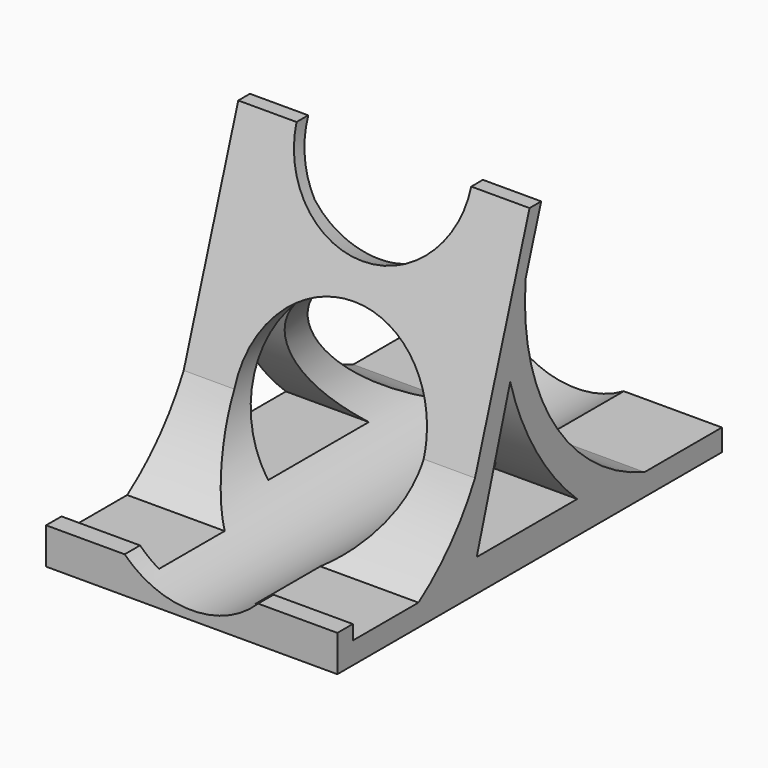
from build123d import *

# Parameters (mm, degrees)
F1_DEPTH = 127
F2_DEPTH = 127
F3_DEPTH = 127
F4_DEPTH = 127
F5_DEPTH = 127
F7_DEPTH = 114.3
F9_DEPTH = 215.9


# Not quite as in the source:
# - a feature names something its author has since deleted; it is built from what else it names


with BuildPart() as f1:
    # F0 (on Right) → F1 (new body)
    with BuildSketch(Plane.YZ):
        Polygon((-23.5780230826, -53.0224030194), (-17.2280230826, -53.0224030194), (15.5594434607, 47.8870429867), (23.9793931173, 73.8009834286), (17.6293931173, 73.8009834286), (-12.109174605, -17.7249168697), align=None)
        Polygon((-80.7280230826, -53.0224030194), (-80.7280230826, -62.5474030194), (122.4719769174, -62.5474030194), (122.4719769174, -53.0224030194), (80.3280323744, -53.0224030194), (-17.2280230826, -53.0224030194), (-23.5780230826, -53.0224030194), (-42.9109744728, -53.0224030194), (-78.7108764052, -53.0224030194), align=None)
    extrude(amount=F1_DEPTH)

    # F0 (on Right) → F2 (join)
    with BuildSketch(Plane.YZ):
        with BuildLine():
            Line((-17.2280230826, -53.0224030194), (80.3280323744, -53.0224030194))
            ThreePointArc((80.3280323744, -53.0224030194), (30.5185291001, -13.7520262922), (15.5594434607, 47.8870429867))
            Line((15.5594434607, 47.8870429867), (-17.2280230826, -53.0224030194))
        make_face()
        with BuildLine():
            Line((-11.1604323611, -48.4367646277), (7.0909718052, 11.3872801885))
            ThreePointArc((7.0909718052, 11.3872801885), (21.2331642185, -21.0320576084), (43.5937792063, -48.4367646277))
            Line((43.5937792063, -48.4367646277), (-11.1604323611, -48.4367646277))
        make_face(mode=Mode.SUBTRACT)
    extrude(amount=F2_DEPTH)

    # F0 (on Right) → F3 (cut)
    with BuildSketch(Plane.YZ):
        with BuildLine():
            ThreePointArc((43.5937792063, -48.4367646277), (21.2331642185, -21.0320576084), (7.0909718052, 11.3872801885))
            Line((7.0909718052, 11.3872801885), (-11.1604323611, -48.4367646277))
            Line((-11.1604323611, -48.4367646277), (43.5937792063, -48.4367646277))
        make_face()
    extrude(amount=-F3_DEPTH, mode=Mode.SUBTRACT)

    # F0 (on Right) → F4 (join)
    with BuildSketch(Plane.YZ):
        with BuildLine():
            ThreePointArc((-12.109174605, -17.7249168697), (-25.2658938129, -37.3320091963), (-42.9109744728, -53.0224030194))
            Line((-42.9109744728, -53.0224030194), (-23.5780230826, -53.0224030194))
            Line((-23.5780230826, -53.0224030194), (-12.109174605, -17.7249168697))
        make_face()
    extrude(amount=F4_DEPTH)

    # F0 (on Right) → F5 (join)
    with BuildSketch(Plane.YZ):
        Polygon((-87.1128812432, -62.5474030194), (-80.7280230826, -62.5474030194), (-80.7280230826, -53.0224030194), (-78.7108764052, -53.0224030194), (-78.7108764052, -46.6724030194), (-87.1128812432, -46.6724030194), align=None)
    extrude(amount=F5_DEPTH)

    # F6 (on face) → F7 (cut)
    with BuildSketch(Plane(origin=(0, -5.7436289571, 1.866218176), x_dir=(1, 0, 0), z_dir=(0, -0.9510565163, 0.3090169944))):
        with BuildLine():
            ThreePointArc((25.4, 75.6366882725), (63.5, 37.5366882725), (101.6, 75.6366882725))
            Line((101.6, 75.6366882725), (25.4, 75.6366882725))
        make_face()
        with BuildLine():
            Line((25.4, 75.6366882725), (101.6, 75.6366882725))
            ThreePointArc((101.6, 75.6366882725), (63.5, 113.7366882725), (25.4, 75.6366882725))
        make_face()
    extrude(amount=-F7_DEPTH, mode=Mode.SUBTRACT)

    # F8 (on face) → F9 (cut)
    with BuildSketch(Plane.XZ.offset(87.1128812432)):
        with BuildLine():
            Line((92.459596055, -46.6724030194), (34.2501482793, -46.6724030194))
            ThreePointArc((34.2501482793, -46.6724030194), (63.3548721671, -58.6806869), (92.459596055, -46.6724030194))
        make_face()
        with BuildLine():
            ThreePointArc((92.459596055, -46.6724030194), (101.4660457483, -33.2538436782), (104.6298721671, -17.4056869))
            ThreePointArc((104.6298721671, -17.4056869), (47.506715389, 20.7054866812), (34.2501482793, -46.6724030194))
            Line((34.2501482793, -46.6724030194), (92.459596055, -46.6724030194))
        make_face()
    extrude(amount=-F9_DEPTH, mode=Mode.SUBTRACT)


solid = f1.part
